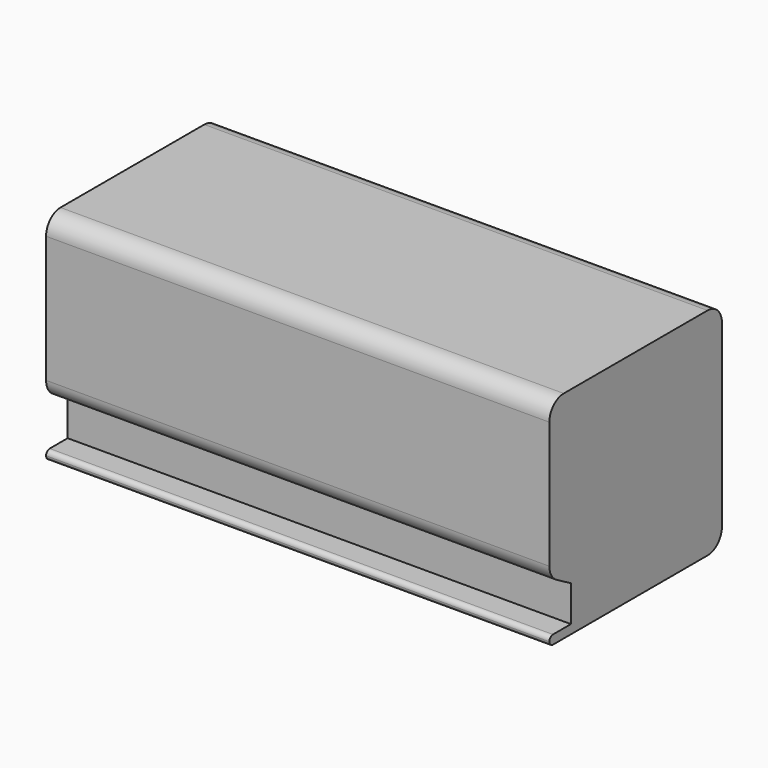
from build123d import *

# Parameters (mm, degrees)
F1_DEPTH = 177.8
F2_R     = 12.7
F3_R     = 3.17499


# Not quite as in the source:
# - a fillet or chamfer is up to 0.001 mm smaller than in the source, because OpenCascade refuses the exact size


with BuildPart() as f1:
    # F0 (on Right) → F1 (new body, symmetric)
    with BuildSketch(Plane.YZ):
        Polygon((70.9975426912, -81.0872844047), (70.9975426912, 71.3127155953), (-81.4024573088, 71.3127155953), (-81.4024573088, -38.3387617767), (-62.3524573088, -49.3372844047), (-62.3524573088, -74.7372844047), (-81.4024573088, -74.7372844047), (-81.4024573088, -81.0872844047), align=None)
    extrude(amount=F1_DEPTH, both=True)

    # F2
    f2_edges = [f1.edges().sort_by_distance(p)[0] for p in [
        (0, -81.402457, -38.338762),
        (0, -81.402457, 71.312716),
        (0, 70.997543, 71.312716),
        (0, 70.997543, -81.087284),
    ]]
    fillet(f2_edges, radius=F2_R)

    # F3 (radius 3.175 in the source; OpenCascade refuses exactly that, so slightly less here)
    f3_edges = [f1.edges().sort_by_distance(p)[0] for p in [
        (0, -81.402457, -74.737284),
        (0, -81.402457, -81.087284),
    ]]
    fillet(f3_edges, radius=F3_R)


solid = f1.part
